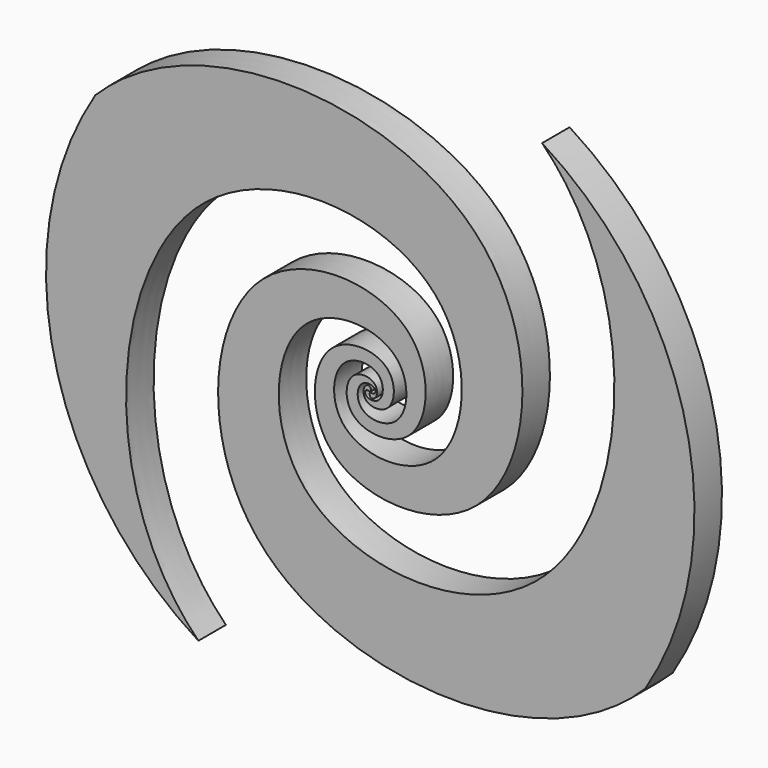
from build123d import *

# Parameters (mm, degrees)
F6_DEPTH = 203.2
F7_COUNT = 2


# Not quite as in the source:
# - the dataset's text gives a spline's control points without its knots; the knots are read off the source's solid


with BuildPart() as f6:
    # F5 (on Front) → F6 (new body)
    with BuildSketch(Plane.XZ):
        with BuildLine():
            add(Edge.make_bspline(
                [(0, 0), (7.4392439626, -4.0425355545), (29.7718987547, -6.6876514062), (32.2888548874, 15.4952437331), (27.1419803188, 23.1823739874)],
                knots=[0, 0, 0, 0, 0.0243427352, 0.04646655, 0.04646655, 0.04646655, 0.04646655], degree=3))
            add(Edge.make_bspline(
                [(0, 0), (-4.0425355545, -7.4392439626), (-6.6876514062, -29.7718987547), (15.4952437331, -32.2888548874), (23.1823739874, -27.1419803188)],
                knots=[0, 0, 0, 0, 0.0243427352, 0.04646655, 0.04646655, 0.04646655, 0.04646655], degree=3))
            add(Edge.make_bspline(
                [(23.1823739874, -27.1419803188), (23.9445462712, -26.5946526707), (24.684729633, -26.0142013139), (25.4, -25.4)],
                knots=[0.0814641628, 0.0814641628, 0.0814641628, 0.0814641628, 0.0831112967, 0.0831112967, 0.0831112967, 0.0831112967], degree=3))
            add(Edge.make_bspline(
                [(25.4, -25.4), (35.8082021572, -15.8609738597), (38.0340418298, 8.0148095006), (27.1419803188, 23.1823739874)],
                knots=[0.0486854704, 0.0486854704, 0.0486854704, 0.0486854704, 0.0814641628, 0.0814641628, 0.0814641628, 0.0814641628], degree=3))
        make_face()
        with BuildLine():
            add(Edge.make_bspline(
                [(27.1419803188, 23.1823739874), (26.6257716321, 23.9533590502), (26.0457347411, 24.6954272662), (25.4, 25.4)],
                knots=[0.04646655, 0.04646655, 0.04646655, 0.04646655, 0.0486854704, 0.0486854704, 0.0486854704, 0.0486854704], degree=3))
            add(Edge.make_bspline(
                [(25.4, -25.4), (35.8082021572, -15.8609738597), (38.0340418298, 8.0148095006), (27.1419803188, 23.1823739874)],
                knots=[0.0486854704, 0.0486854704, 0.0486854704, 0.0486854704, 0.0814641628, 0.0814641628, 0.0814641628, 0.0814641628], degree=3))
            add(Edge.make_bspline(
                [(25.4, -25.4), (43.7092818518, -9.6778542385), (48.257421986, 77.0054874262), (-144.243671066, 88.8728103608), (-162.6559135138, -221.2563261174), (340.2839751081, -251.5411782008), (387.9840127558, 561.6202835846), (-922.9801498647, 639.085188427), (-1075.785700849, -1482.2240141172), (1016, -1625.6), (1625.6, -1016)],
                knots=[0.0831112967, 0.0831112967, 0.0831112967, 0.0831112967, 0.1252741509, 0.1797061616, 0.2485578142, 0.3363267943, 0.447879221, 0.5898205391, 0.7703510952, 1, 1, 1, 1], degree=3))
            ThreePointArc((1625.6, -1016), (1867.8932731824, 431.0522938113), (1016, 1625.6))
            add(Edge.make_bspline(
                [(25.4, 25.4), (9.6778542385, 43.7092818518), (-77.0054874262, 48.257421986), (-88.8728103608, -144.243671066), (221.2563261174, -162.6559135138), (251.5411782008, 340.2839751081), (-561.6202835846, 387.9840127558), (-639.085188427, -922.9801498647), (1482.2240141172, -1075.785700849), (1625.6, 1016), (1016, 1625.6)],
                knots=[0.0831112967, 0.0831112967, 0.0831112967, 0.0831112967, 0.1252741509, 0.1797061616, 0.2485578142, 0.3363267943, 0.447879221, 0.5898205391, 0.7703510952, 1, 1, 1, 1], degree=3))
        make_face()
    extrude(amount=F6_DEPTH)


with BuildPart() as f7_1:
    # F7: instance of F6
    add(f6.part.rotate(Axis((0, 0, 0), (0, 1, 0)), 1 * 360 / F7_COUNT))


solid = Compound([f6.part, f7_1.part])
